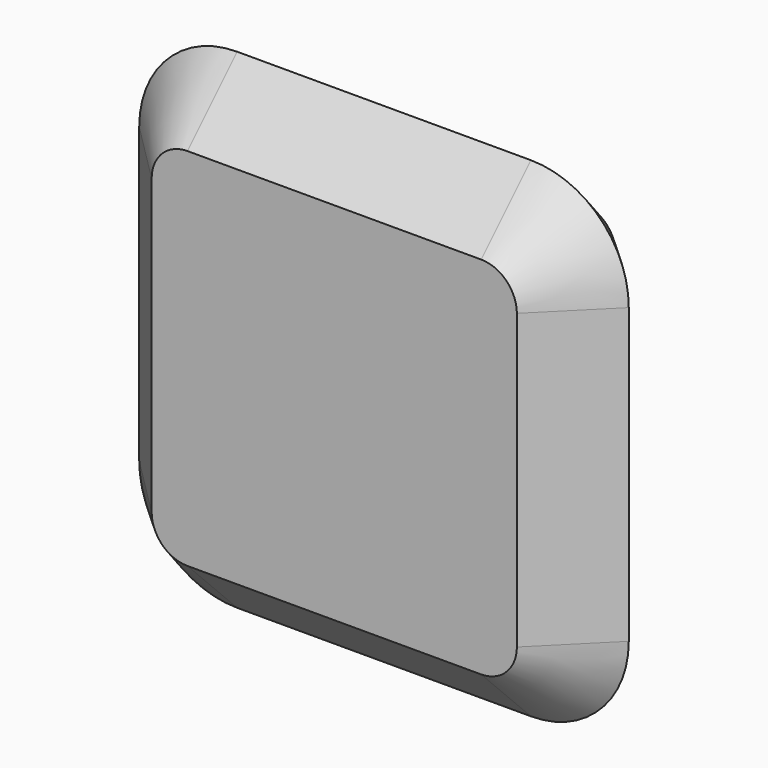
from build123d import *

# Parameters (mm, degrees)
F1_DEPTH = 25.4
F2_SIZE  = 12.69999


# Not quite as in the source:
# - a fillet or chamfer is up to 0.001 mm smaller than in the source, because OpenCascade refuses the exact size


with BuildPart() as f1:
    # F0 (on Front) → F1 (new body)
    with BuildSketch(Plane.XZ):
        with BuildLine():
            Line((-30, -50), (30, -50))
            ThreePointArc((30, -50), (44.1421356237, -44.1421356237), (50, -30))
            Line((50, -30), (50, 30))
            ThreePointArc((50, 30), (44.1421356237, 44.1421356237), (30, 50))
            Line((30, 50), (-30, 50))
            ThreePointArc((-30, 50), (-44.1421356237, 44.1421356237), (-50, 30))
            Line((-50, 30), (-50, -30))
            ThreePointArc((-50, -30), (-44.1421356237, -44.1421356237), (-30, -50))
        make_face()
    extrude(amount=F1_DEPTH)

    # F2 (size 12.7 in the source; OpenCascade refuses exactly that, so slightly less here)
    f2_edges = [f1.edges().sort_by_distance(p)[0] for p in [
        (-44.142136, -25.4, -44.142136),
        (0, -25.4, -50),
        (44.142136, -25.4, -44.142136),
        (50, -25.4, 0),
        (44.142136, -25.4, 44.142136),
        (0, -25.4, 50),
        (-44.142136, -25.4, 44.142136),
        (-50, -25.4, 0),
        (-44.142136, 0, -44.142136),
        (0, 0, -50),
        (44.142136, 0, -44.142136),
        (50, 0, 0),
        (44.142136, 0, 44.142136),
        (0, 0, 50),
        (-44.142136, 0, 44.142136),
        (-50, 0, 0),
    ]]
    chamfer(f2_edges, length=F2_SIZE)


solid = f1.part
